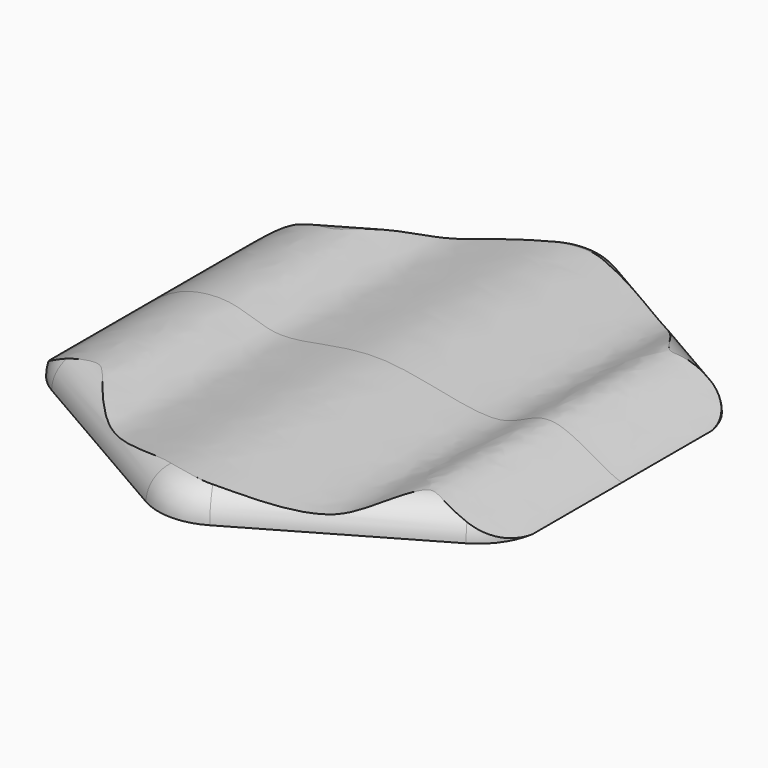
from build123d import *

# Parameters (mm, degrees)
F1_DEPTH      = 100
F2_R          = 200
F3_R          = 99.99999
F5_DEPTH      = 1500
F5_DEPTH_BACK = 1500


# Not quite as in the source:
# - a fillet or chamfer is up to 0.001 mm smaller than in the source, because OpenCascade refuses the exact size


with BuildPart() as f1:
    # F0 (on Top) → F1 (new body)
    with BuildSketch(Plane.XY):
        Polygon((750, -433.0127018922), (750, 433.0127018922), (0, 866.0254037844), (-750, 433.0127018922), (-750, -433.0127018922), (0, -866.0254037844), align=None)
    extrude(amount=F1_DEPTH)

    # F2
    f2_edges = [f1.edges().sort_by_distance(p)[0] for p in [
        (0, -866.025404, 50),
        (750, -433.012702, 50),
        (750, 433.012702, 50),
        (0, 866.025404, 50),
        (-750, -433.012702, 50),
        (-750, 433.012702, 50),
    ]]
    fillet(f2_edges, radius=F2_R)

    # F3 (radius 100 in the source; OpenCascade refuses exactly that, so slightly less here)
    f3_edges = [f1.edges().sort_by_distance(p)[0] for p in [
        (750, 0, 100),
        (723.205081, -417.542648, 100),
        (723.205081, 417.542648, 100),
        (375, -649.519053, 100),
        (375, 649.519053, 100),
        (0, -835.085296, 100),
        (0, 835.085296, 100),
        (-375, -649.519053, 100),
        (-375, 649.519053, 100),
        (-723.205081, -417.542648, 100),
        (-723.205081, 417.542648, 100),
        (-750, 0, 100),
    ]]
    fillet(f3_edges, radius=F3_R)

    # F4 (on Front) → F5 (cut, two sides)
    with BuildSketch(Plane.XZ) as f5_sk:
        with BuildLine():
            Line((-753.6191940308, 173.2049435377), (-753.6191940308, 0))
            add(Edge.make_bspline(
                [(-753.6191940308, 0), (-718.3231692767, 29.2561861316), (-644.6494451981, 90.3228983088), (-466.3614283566, 111.8904392597), (-323.0185815358, 26.7898559926), (-12.6911606495, 145.5553533179), (375.6182682521, -7.5667455139), (520.8266428701, 161.9796860109), (809.3143182693, -82.3282923815), (772.5314440442, 78.0143531888), (756.3662528992, 148.4811007977)],
                knots=[0, 0, 0, 0, 0.1024364089, 0.2138164786, 0.3203190993, 0.4747377435, 0.6448171558, 0.7594948982, 0.8943037752, 1, 1, 1, 1], degree=3))
            Line((756.3662528992, 148.4811007977), (-753.6191940308, 173.2049435377))
        make_face()
    extrude(amount=F5_DEPTH, mode=Mode.SUBTRACT)
    extrude(f5_sk.sketch, amount=-F5_DEPTH_BACK, mode=Mode.SUBTRACT)


solid = f1.part
